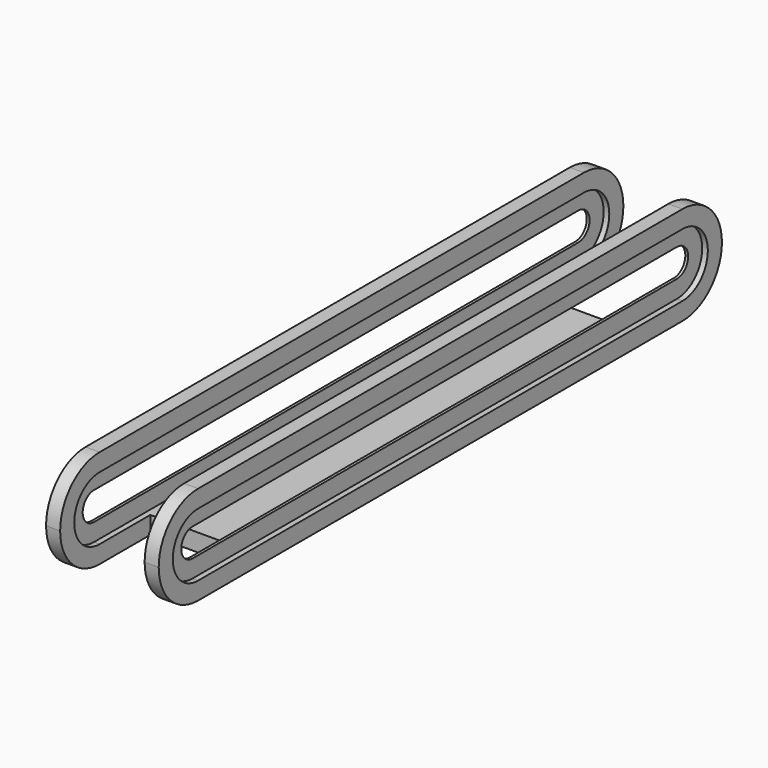
from build123d import *

# Parameters (mm, degrees)
F1_DEPTH      = 125
F1_DEPTH_BACK = 125
F6_DEPTH      = 5.0009999999
F7_DEPTH      = 5.0010000001
F8_DEPTH      = 2
F9_DEPTH      = 2
F10_DEPTH     = 2
F11_DEPTH     = 2
F12_W         = 30
F12_H         = 40
F13_DEPTH     = 35.001
F14_R         = 17.49999


# Not quite as in the source:
# - a fillet or chamfer is up to 0.001 mm smaller than in the source, because OpenCascade refuses the exact size


with BuildPart() as f1:
    # F0 (on Front) → F1 (new body, two sides)
    with BuildSketch(Plane.XZ) as f1_sk:
        Polygon((-20, -17.5), (20, -17.5), (20, 17.5), (15, 17.5), (15, -11.25), (-15, -11.25), (-15, 17.5), (-20, 17.5), align=None)
    extrude(amount=F1_DEPTH)
    extrude(f1_sk.sketch, amount=-F1_DEPTH_BACK)

    # F3 (on face) → F6 (cut, through all)
    with BuildSketch(Plane(origin=(15.0000000001, 0, 0), x_dir=(0, -1, 0), z_dir=(-1, 0, 0))):
        with BuildLine():
            Line((107.5, 4.9999999999), (0, 4.9999999999))
            Line((0, 4.9999999999), (-107.5, 4.9999999999))
            ThreePointArc((-107.5, 4.9999999999), (-112.5, -2e-10), (-107.5, -5.0000000004))
            Line((-107.5, -5.0000000004), (0, -5.0000000004))
            Line((0, -5.0000000004), (107.5, -5.0000000004))
            ThreePointArc((107.5, -5.0000000004), (112.5000000001, -2e-10), (107.5, 4.9999999999))
        make_face()
    extrude(amount=-F6_DEPTH, mode=Mode.SUBTRACT)

    # F2 (on face) → F7 (cut, through all)
    with BuildSketch(Plane.YZ.offset(-14.9999999999)):
        with BuildLine():
            Line((107.5, 5), (0, 5))
            Line((0, 5), (-107.5, 5))
            ThreePointArc((-107.5, 5), (-112.5, 0), (-107.5, -5))
            Line((-107.5, -5), (0, -5))
            Line((0, -5), (107.5, -5))
            ThreePointArc((107.5, -5), (112.5, 0), (107.5, 5))
        make_face()
    extrude(amount=-F7_DEPTH, mode=Mode.SUBTRACT)

    # F3 (on face) → F8 (cut)
    with BuildSketch(Plane(origin=(15.0000000001, 0, 0), x_dir=(0, -1, 0), z_dir=(-1, 0, 0))):
        with BuildLine():
            Line((107.5, 11.25), (0, 11.25))
            Line((0, 11.25), (-107.5, 11.25))
            ThreePointArc((-107.5, 11.25), (-118.7500000002, -2e-10), (-107.5, -11.2500000005))
            Line((-107.5, -11.2500000005), (0, -11.2500000005))
            Line((0, -11.2500000005), (107.5, -11.2500000005))
            ThreePointArc((107.5, -11.2500000005), (118.7500000002, -2e-10), (107.5, 11.25))
        make_face()
        with BuildLine():
            Line((-107.5, 4.9999999999), (0, 4.9999999999))
            Line((0, 4.9999999999), (107.5, 4.9999999999))
            ThreePointArc((107.5, 4.9999999999), (112.5000000001, -2e-10), (107.5, -5.0000000004))
            Line((107.5, -5.0000000004), (0, -5.0000000004))
            Line((0, -5.0000000004), (-107.5, -5.0000000004))
            ThreePointArc((-107.5, -5.0000000004), (-112.5, -2e-10), (-107.5, 4.9999999999))
        make_face(mode=Mode.SUBTRACT)
    extrude(amount=-F8_DEPTH, mode=Mode.SUBTRACT)

    # F2 (on face) → F9 (cut)
    with BuildSketch(Plane.YZ.offset(-14.9999999999)):
        with BuildLine():
            Line((107.5, 11.25), (0, 11.25))
            Line((0, 11.25), (-107.5, 11.25))
            ThreePointArc((-107.5, 11.25), (-118.75, 0), (-107.5, -11.25))
            Line((-107.5, -11.25), (0, -11.25))
            Line((0, -11.25), (107.5, -11.25))
            ThreePointArc((107.5, -11.25), (118.75, 0), (107.5, 11.25))
        make_face()
        with BuildLine():
            Line((-107.5, 5), (0, 5))
            Line((0, 5), (107.5, 5))
            ThreePointArc((107.5, 5), (112.5, 0), (107.5, -5))
            Line((107.5, -5), (0, -5))
            Line((0, -5), (-107.5, -5))
            ThreePointArc((-107.5, -5), (-112.5, 0), (-107.5, 5))
        make_face(mode=Mode.SUBTRACT)
    extrude(amount=-F9_DEPTH, mode=Mode.SUBTRACT)

    # F4 (on face) → F10 (cut)
    with BuildSketch(Plane(origin=(-20, 0, 1e-10), x_dir=(0, -1, 0), z_dir=(-1, 0, 0))):
        with BuildLine():
            Line((107.5, 11.25), (0, 11.25))
            Line((0, 11.25), (-107.5, 11.25))
            ThreePointArc((-107.5, 11.25), (-118.75, 0), (-107.5, -11.25))
            Line((-107.5, -11.25), (0, -11.25))
            Line((0, -11.25), (107.5, -11.25))
            ThreePointArc((107.5, -11.25), (118.75, 0), (107.5, 11.25))
        make_face()
        with BuildLine():
            Line((-107.5, 5), (0, 5))
            Line((0, 5), (107.5, 5))
            ThreePointArc((107.5, 5), (112.5, 0), (107.5, -5))
            Line((107.5, -5), (0, -5))
            Line((0, -5), (-107.5, -5))
            ThreePointArc((-107.5, -5), (-112.5, 0), (-107.5, 5))
        make_face(mode=Mode.SUBTRACT)
    extrude(amount=-F10_DEPTH, mode=Mode.SUBTRACT)

    # F5 (on face) → F11 (cut)
    with BuildSketch(Plane.YZ.offset(20)):
        with BuildLine():
            Line((107.5, 11.25), (0, 11.25))
            Line((0, 11.25), (-107.5, 11.25))
            ThreePointArc((-107.5, 11.25), (-118.75, 0), (-107.5, -11.25))
            Line((-107.5, -11.25), (0, -11.25))
            Line((0, -11.25), (107.5, -11.25))
            ThreePointArc((107.5, -11.25), (118.75, 0), (107.5, 11.25))
        make_face()
        with BuildLine():
            Line((-107.5, 5), (0, 5))
            Line((0, 5), (107.5, 5))
            ThreePointArc((107.5, 5), (112.5, 0), (107.5, -5))
            Line((107.5, -5), (0, -5))
            Line((0, -5), (-107.5, -5))
            ThreePointArc((-107.5, -5), (-112.5, 0), (-107.5, 5))
        make_face(mode=Mode.SUBTRACT)
    extrude(amount=-F11_DEPTH, mode=Mode.SUBTRACT)

    # F12 (on face) → F13 (cut, through all)
    with BuildSketch(Plane(origin=(0, 0, -17.5), x_dir=(1, 0, 0), z_dir=(0, 0, -1))):
        with Locations((-2e-10, -105)):
            Rectangle(F12_W, F12_H)
        with Locations((-2e-10, 105)):
            Rectangle(F12_W, F12_H)
    extrude(amount=-F13_DEPTH, mode=Mode.SUBTRACT)

    # F14 (radius 17.5 in the source; OpenCascade refuses exactly that, so slightly less here)
    f14_edges = [f1.edges().sort_by_distance(p)[0] for p in [
        (17.5, 125, 17.5),
        (17.5, 125, -17.5),
        (-17.5, 125, -17.5),
        (-17.5, 125, 17.5),
        (-17.5, -125, -17.5),
        (-17.5, -125, 17.5),
        (17.5, -125, 17.5),
        (17.5, -125, -17.5),
    ]]
    fillet(f14_edges, radius=F14_R)


solid = f1.part
